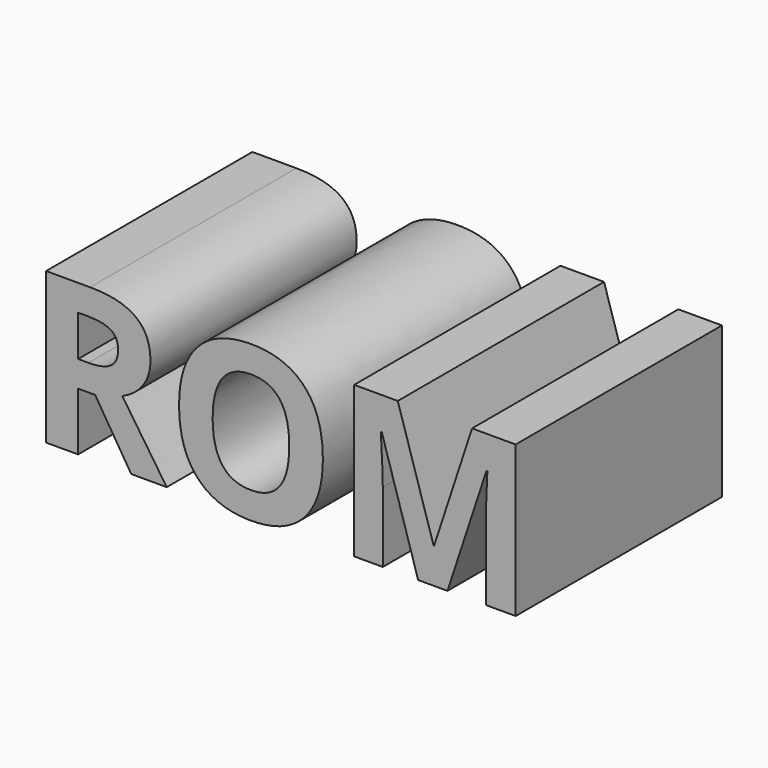
from build123d import *

# Parameters (mm, degrees)
F0_TEXT_SIZE = 8.205909029
F1_DEPTH     = 10
F2_DEPTH     = 10


# Not quite as in the source:
# - Text() gives the source's letters only with a copy of the font that has no kerning and outlines rounded to 1/6400 em; it was checked with that copy


with BuildPart() as f1:
    # F0 (on Front) → F1 (new body)
    with BuildSketch(Plane.XZ):
        with Locations((-19.480058731, 0)):
            Text('ROM', F0_TEXT_SIZE, font='Open Sans', font_style=FontStyle.BOLD, text_align=(TextAlign.LEFT, TextAlign.BOTTOM))
    extrude(amount=F1_DEPTH)


with BuildPart() as f2:
    # F0 (on Front) → F2 (new body)
    with BuildSketch(Plane.XZ):
        with Locations((-19.480058731, 0)):
            Text('ROM', F0_TEXT_SIZE, font='Open Sans', font_style=FontStyle.BOLD, text_align=(TextAlign.LEFT, TextAlign.BOTTOM))
    extrude(amount=F2_DEPTH)


solid = Compound([f1.part, f2.part])
